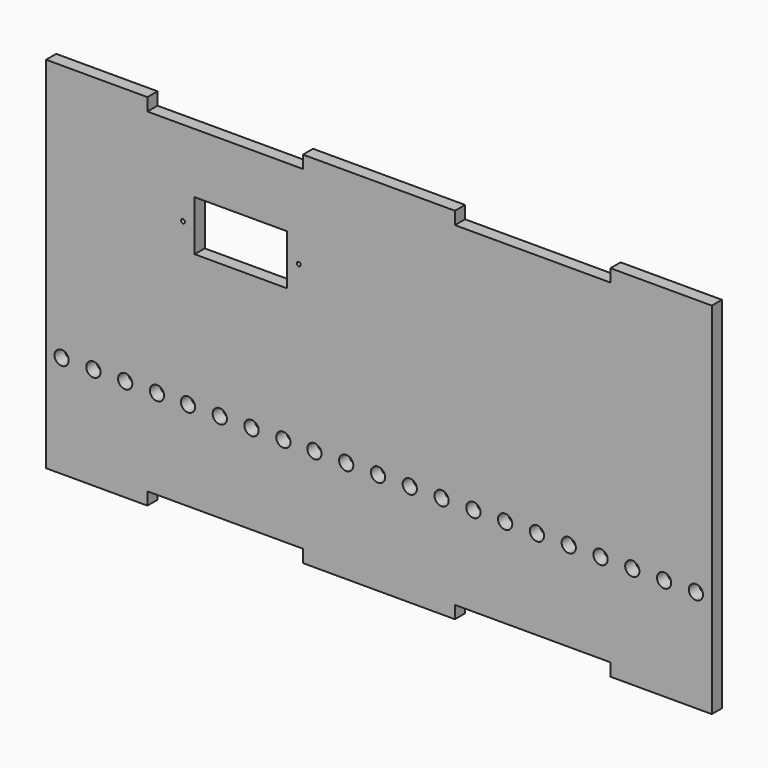
from build123d import *

# Parameters (mm, degrees)
F0_W     = 25.4
F0_H     = 3.175
F0_W_2   = 38.1
F0_R     = 1.7859375
F0_R_2   = 0.5
F1_DEPTH = 3.175


# Not quite as in the source:
# - a length typed as a fraction of an inch, garbled in the dataset ("3 / 203.2 mm" for 3/8 in), is restored


with BuildPart() as f1:
    # F0 (on Front) → F1 (new body)
    with BuildSketch(Plane.XZ):
        with Locations((-54.5774, 62.9375024)):
            Rectangle(F0_W, F0_H)
        with Locations((16.1738, 62.9375024)):
            Rectangle(F0_W_2, F0_H)
        with Locations((86.925, 62.9375024)):
            Rectangle(F0_W, F0_H)
        with Locations((86.925, -24.0574976)):
            Rectangle(F0_W, F0_H)
        with Locations((16.1738, -24.0574976)):
            Rectangle(F0_W_2, F0_H)
        with Locations((-54.5774, -24.0574976)):
            Rectangle(F0_W, F0_H)
        Polygon((-67.2774, 61.1329712169), (-67.2774, -22.4699976), (-41.8774, -22.4699976), (-2.8762, -22.4699976), (35.2238, -22.4699976), (74.225, -22.4699976), (99.625, -22.4699976), (99.625, 61.3500024), (74.225, 61.3500024), (35.2238, 61.3500024), (-2.8762, 61.3500024), (-41.8774, 61.3500024), (-67.2774, 61.3500024), align=None)
        with Locations((-63.3824, 0)):
            Circle(F0_R, mode=Mode.SUBTRACT)
        with Locations((-55.4124, 0)):
            Circle(F0_R, mode=Mode.SUBTRACT)
        with Locations((-47.4424, 0)):
            Circle(F0_R, mode=Mode.SUBTRACT)
        with Locations((-39.4724, 0)):
            Circle(F0_R, mode=Mode.SUBTRACT)
        with Locations((-31.7, 0)):
            Circle(F0_R, mode=Mode.SUBTRACT)
        with Locations((-23.73, 0)):
            Circle(F0_R, mode=Mode.SUBTRACT)
        with Locations((-15.76, 0)):
            Circle(F0_R, mode=Mode.SUBTRACT)
        with Locations((-7.79, 0)):
            Circle(F0_R, mode=Mode.SUBTRACT)
        Circle(F0_R, mode=Mode.SUBTRACT)
        with Locations((7.97, 0)):
            Circle(F0_R, mode=Mode.SUBTRACT)
        with Locations((15.94, 0)):
            Circle(F0_R, mode=Mode.SUBTRACT)
        with Locations((23.91, 0)):
            Circle(F0_R, mode=Mode.SUBTRACT)
        with Locations((31.88, 0)):
            Circle(F0_R, mode=Mode.SUBTRACT)
        with Locations((39.85, 0)):
            Circle(F0_R, mode=Mode.SUBTRACT)
        with Locations((47.82, 0)):
            Circle(F0_R, mode=Mode.SUBTRACT)
        with Locations((55.79, 0)):
            Circle(F0_R, mode=Mode.SUBTRACT)
        with Locations((63.76, 0)):
            Circle(F0_R, mode=Mode.SUBTRACT)
        with Locations((71.73, 0)):
            Circle(F0_R, mode=Mode.SUBTRACT)
        with Locations((79.7, 0)):
            Circle(F0_R, mode=Mode.SUBTRACT)
        with Locations((87.67, 0)):
            Circle(F0_R, mode=Mode.SUBTRACT)
        with Locations((95.64, 0)):
            Circle(F0_R, mode=Mode.SUBTRACT)
        with Locations((-32.93, 40.005)):
            Circle(F0_R_2, mode=Mode.SUBTRACT)
        Polygon((-30.03, 33.705), (-30.03, 46.305), (-18.43, 46.305), (-6.83, 46.305), (-6.83, 33.705), (-18.43, 33.705), align=None, mode=Mode.SUBTRACT)
        with Locations((-3.93, 40.005)):
            Circle(F0_R_2, mode=Mode.SUBTRACT)
    extrude(amount=F1_DEPTH)


solid = f1.part
